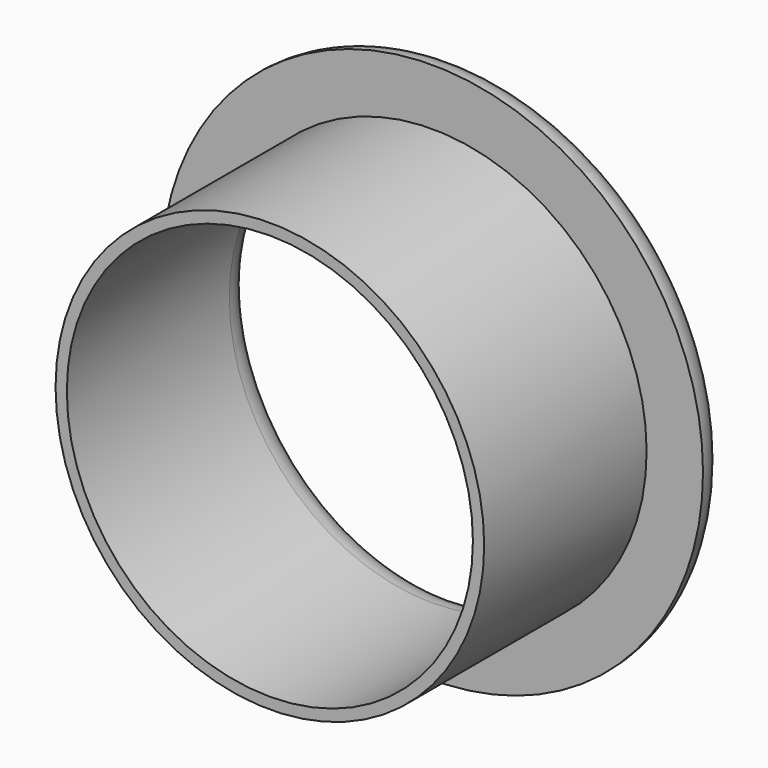
from build123d import *

# Parameters (mm, degrees)
F0_R     = 24
F1_DEPTH = 3
F2_R     = 19
F3_DEPTH = 18
F5_D     = 36
F6_R     = 2.99999


# Not quite as in the source:
# - a fillet or chamfer is up to 0.001 mm smaller than in the source, because OpenCascade refuses the exact size


with BuildPart() as f1:
    # F0 (on Front) → F1 (new body)
    with BuildSketch(Plane.XZ):
        Circle(F0_R)
    extrude(amount=F1_DEPTH)

    # F2 (on face) → F3 (join)
    with BuildSketch(Plane.XZ.offset(3)):
        Circle(F2_R)
    extrude(amount=F3_DEPTH)

    # F5 (through all)
    with Locations(Plane(origin=(0, 0, 0), x_dir=(-1, 0, 0), z_dir=(0, 1, 0))):
        with Locations((0, 0)):
            Hole(F5_D / 2)

    # F6 (radius 3 in the source; OpenCascade refuses exactly that, so slightly less here)
    f6_edges = [f1.edges().sort_by_distance(p)[0] for p in [
        (-24, 0, 0),
        (18, 0, 0),
    ]]
    fillet(f6_edges, radius=F6_R)


solid = f1.part
